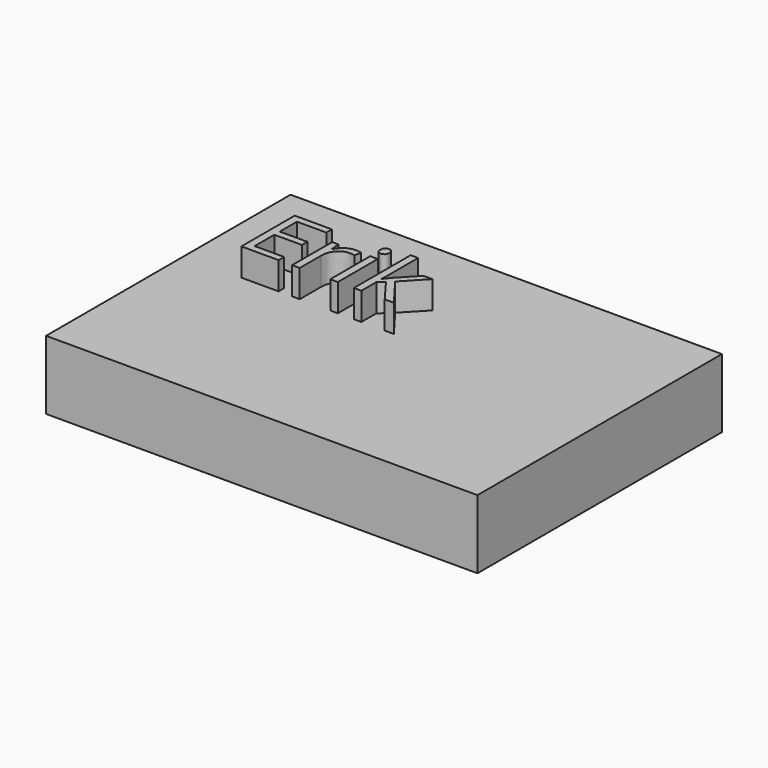
from build123d import *

# Parameters (mm, degrees)
F0_W         = 31.3507141545
F0_H         = 22.2067544237
F1_DEPTH     = 5
F2_TEXT_SIZE = 6.7838079606
F3_DEPTH     = 2


# Not quite as in the source:
# - a feature names something its author has since deleted; it is built from what else it names
# - Text() gives the source's letters only with a copy of the font that has no kerning and outlines rounded to 1/6400 em; it was checked with that copy


with BuildPart() as f1:
    # F0 (on Top) → F1 (new body)
    with BuildSketch(Plane.XY):
        with Locations((-1.8661129288, -1.3995855115)):
            Rectangle(F0_W, F0_H)
    extrude(amount=F1_DEPTH)

    # F2 (on face) → F3 (join)
    with BuildSketch(Plane.XY.offset(5)):
        with Locations((-14.0150357038, 0)):
            Text('Erik', F2_TEXT_SIZE, font='Open Sans', text_align=(TextAlign.LEFT, TextAlign.BOTTOM))
    extrude(amount=F3_DEPTH)


solid = f1.part
